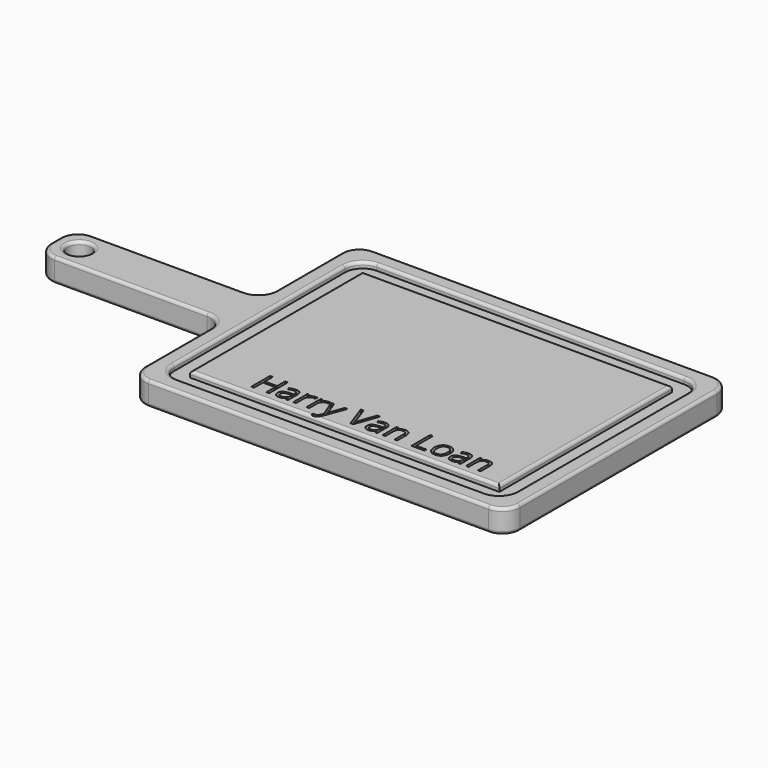
from build123d import *

# Parameters (mm, degrees)
F0_W         = 203.2
F0_H         = 50.8
F1_DEPTH     = 25.4
F2_R         = 12.7
F3_DEPTH     = 25.4
F5_DEPTH     = 6.35
F6_R         = 19.05
F7_R         = 3.175
F8_TEXT_SIZE = 35.3937599338
F9_DEPTH     = 5.08


# Not quite as in the source:
# - Text() gives the source's letters only with a copy of the font that has no kerning and outlines rounded to 1/6400 em; it was checked with that copy


with BuildPart() as f1:
    # F0 (on Top) → F1 (new body)
    with BuildSketch(Plane.XY):
        Polygon((0, 127), (0, 0), (406.4, 0), (406.4, 304.8), (0, 304.8), (0, 177.8), align=None)
        with Locations((-101.6, 152.4)):
            Rectangle(F0_W, F0_H)
    extrude(amount=F1_DEPTH)

    # F2 (on face) → F3 (cut)
    with BuildSketch(Plane.XY.offset(25.4)):
        with Locations((-177.8, 152.4)):
            Circle(F2_R)
    extrude(amount=-F3_DEPTH, mode=Mode.SUBTRACT)

    # F4 (on face) → F5 (cut)
    with BuildSketch(Plane.XY.offset(25.4)):
        Polygon((17.7800021648, 127), (17.7800021648, 17.7800021648), (388.6199978352, 17.7800021648), (388.6199978352, 287.0199978352), (17.7800021648, 287.0199978352), (17.7800021648, 177.8), align=None)
        Polygon((35.5600080967, 127), (35.5600080967, 177.8), (35.5600080967, 269.2399919033), (370.8399919033, 269.2399919033), (370.8399919033, 35.5600080967), (35.5600080967, 35.5600080967), align=None, mode=Mode.SUBTRACT)
    extrude(amount=-F5_DEPTH, mode=Mode.SUBTRACT)

    # F6
    f6_edges = [f1.edges().sort_by_distance(p)[0] for p in [
        (17.780002, 287.019998, 22.225),
        (388.619998, 287.019998, 22.225),
        (388.619998, 17.780002, 22.225),
        (17.780002, 17.780002, 22.225),
        (0, 0, 12.7),
        (0, 127, 12.7),
        (-203.2, 127, 12.7),
        (-203.2, 177.8, 12.7),
        (0, 177.8, 12.7),
        (0, 304.8, 12.7),
        (406.4, 304.8, 12.7),
        (406.4, 0, 12.7),
    ]]
    fillet(f6_edges, radius=F6_R)

    # F7
    f7_edges = [f1.edges().sort_by_distance(p)[0] for p in [
        (203.2, 269.239992, 25.4),
        (370.839992, 152.4, 25.4),
        (203.2, 35.560008, 25.4),
        (35.560008, 152.4, 25.4),
        (0, 63.5, 25.4),
        (-5.579616, 121.420384, 25.4),
        (5.579616, 5.579616, 25.4),
        (-101.6, 127, 25.4),
        (203.2, 0, 25.4),
        (-197.620384, 132.579616, 25.4),
        (400.820384, 5.579616, 25.4),
        (-203.2, 152.4, 25.4),
        (406.4, 152.4, 25.4),
        (-197.620384, 172.220384, 25.4),
        (400.820384, 299.220384, 25.4),
        (-101.6, 177.8, 25.4),
        (203.2, 304.8, 25.4),
        (-5.579616, 183.379616, 25.4),
        (5.579616, 299.220384, 25.4),
        (0, 241.3, 25.4),
        (-190.5, 152.4, 25.4),
        (203.2, 17.780002, 25.4),
        (23.359618, 23.359618, 25.4),
        (383.040382, 23.359618, 25.4),
        (17.780002, 152.4, 25.4),
        (388.619998, 152.4, 25.4),
        (23.359618, 281.440382, 25.4),
        (383.040382, 281.440382, 25.4),
        (203.2, 287.019998, 25.4),
        (0, 63.5, 0),
        (-5.579616, 121.420384, 0),
        (5.579616, 5.579616, 0),
        (-101.6, 127, 0),
        (203.2, 0, 0),
        (-197.620384, 132.579616, 0),
        (400.820384, 5.579616, 0),
        (-203.2, 152.4, 0),
        (406.4, 152.4, 0),
        (-197.620384, 172.220384, 0),
        (400.820384, 299.220384, 0),
        (-101.6, 177.8, 0),
        (203.2, 304.8, 0),
        (-5.579616, 183.379616, 0),
        (5.579616, 299.220384, 0),
        (0, 241.3, 0),
        (-190.5, 152.4, 0),
    ]]
    fillet(f7_edges, radius=F7_R)

    # F8 (on face) → F9 (cut)
    with BuildSketch(Plane.XY.offset(25.4)):
        with Locations((90.8050021648, 45.5322970318)):
            Text('Harry Van Loan', F8_TEXT_SIZE, font='Open Sans', text_align=(TextAlign.LEFT, TextAlign.BOTTOM))
    extrude(amount=-F9_DEPTH, mode=Mode.SUBTRACT)


solid = f1.part
